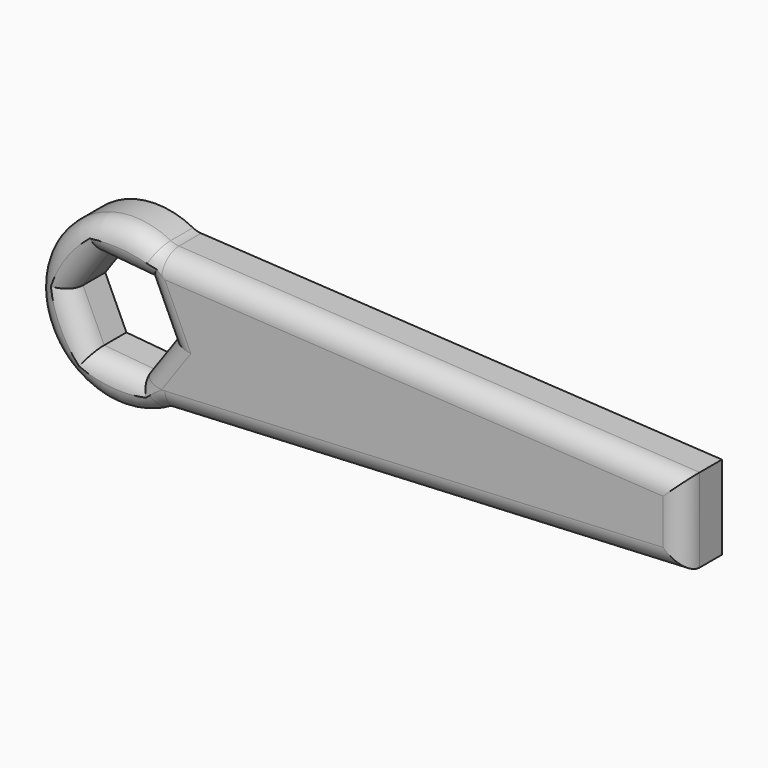
from build123d import *

# Parameters (mm, degrees)
F1_DEPTH      = 11.8
F2_T3_ANGLE   = 23.9952218253
F2_T6_ANGLE   = 236.5757489995
F2_T9_ANGLE   = 26.5092715393
F2_T12_DEPTH  = 139.4367119933
F2_T15_DEPTH  = 45.5289069563
F2_T18_DEPTH  = 140.3160479541
F2_T21_DEPTH  = 37.3901770892
F2_T26_DEPTH  = 37.3901770892
F2_T31_DEPTH  = 37.3901770892
F2_T36_DEPTH  = 37.3901770892
F2_T41_DEPTH  = 37.3901770892
F2_T46_DEPTH  = 37.3901770892
F2_T52_DEPTH  = 37.3901770892
F2_T56_DEPTH  = 37.3901770892
F2_T62_DEPTH  = 37.3901770892
F2_T66_DEPTH  = 37.3901770892
F2_T72_DEPTH  = 37.3901770892
F2_T76_DEPTH  = 37.3901770892
F2_T82_DEPTH  = 37.3901770892
F2_T86_DEPTH  = 37.3901770892
F2_T92_DEPTH  = 37.3901770892
F2_T96_DEPTH  = 37.3901770892
F2_T102_DEPTH = 37.3901770892
F2_T106_DEPTH = 37.3901770892


# Not quite as in the source:
# - a fillet or chamfer that OpenCascade refuses, or shapes differently, is made with other operations: its cross-section is extruded or revolved along the edge and cut away or added


with BuildPart() as f1:
    # F0 (on Front) → F1 (new body)
    with BuildSketch(Plane.XZ):
        with BuildLine():
            ThreePointArc((-45.4681624589, 17.2222085509), (-46.4995658162, 17.3907127083), (-47.4734123647, 17.7699348549))
            ThreePointArc((-47.4734123647, 17.7699348549), (-76.6250444945, -0.3533911925), (-46.8510355825, -17.4349893659))
            ThreePointArc((-46.8510355825, -17.4349893659), (-45.7861203938, -16.9901072457), (-44.6475715962, -16.8012393137))
            Line((-44.6475715962, -16.8012393137), (82.1385234594, -10.6194149703))
            Line((82.1385234594, -10.6194149703), (82.1385234594, 9.909491986))
            Line((82.1385234594, 9.909491986), (-45.4681624589, 17.2222085509))
        make_face()
        Polygon((-49.4849642992, 10.1187057679), (-44.2971102089, -1.1330789012), (-51.4475145251, -11.2517846691), (-63.7857729316, -10.1187057679), (-68.9736270219, 1.1330789012), (-61.8232227057, 11.2517846691), align=None, mode=Mode.SUBTRACT)
    extrude(amount=F1_DEPTH)

    # F2: fillet of radius 5 on 12 edges, made by hand


with BuildPart() as f2_tool1:
    # F2_s2 → F2_t3 (revolve)
    with BuildSketch(Plane(origin=(-46.3030483671, 0, 2.6534743565), x_dir=(0, 1, 0), z_dir=(0.9983620051, 0, -0.0572128202))):
        with BuildLine():
            ThreePointArc((-6.8, 14.5926368593), (-10.3355339059, 13.1281707652), (-11.8, 9.5926368593))
            Line((-11.8, 9.5926368593), (-11.8, 14.5926368593))
            Line((-11.8, 14.5926368593), (-6.8, 14.5926368593))
        make_face()
    revolve(axis=Axis((-45.1820983581, -11.8, 22.2140185763), (0, 1, 0)), revolution_arc=F2_T3_ANGLE)


with BuildPart() as f2_tool4:
    # F2_s5 → F2_t6 (revolve)
    with BuildSketch(Plane(origin=(-44.7416696351, 0, 23.0682455015), x_dir=(0, 1, 0), z_dir=(0.8888167443, 0, -0.4582628013))):
        with BuildLine():
            ThreePointArc((-6.8, -5.9610832949), (-10.3355339059, -7.425549389), (-11.8, -10.9610832949))
            Line((-11.8, -10.9610832949), (-11.8, -5.9610832949))
            Line((-11.8, -5.9610832949), (-6.8, -5.9610832949))
        make_face()
    revolve(axis=Axis((-56.6353686154, -11.8, 0), (0, -1, 0)), revolution_arc=F2_T6_ANGLE)


with BuildPart() as f2_tool7:
    # F2_s8 → F2_t9 (revolve)
    with BuildSketch(Plane(origin=(-43.0708942729, 0, -24.1709337899), x_dir=(0, 1, 0), z_dir=(-0.8720634381, 0, -0.4893928482))):
        with BuildLine():
            ThreePointArc((-6.8, -7.7241449756), (-10.3355339059, -9.1886110696), (-11.8, -12.7241449756))
            Line((-11.8, -12.7241449756), (-11.8, -7.7241449756))
            Line((-11.8, -7.7241449756), (-6.8, -7.7241449756))
        make_face()
    revolve(axis=Axis((-44.4040713414, -11.8, -21.7953065565), (0, 1, 0)), revolution_arc=F2_T9_ANGLE)


with BuildPart() as f2_tool10:
    # F2_s11 → F2_t12 (new body)
    with BuildSketch(Plane(origin=(-45.3589315248, 0, -2.2116064618), x_dir=(0, 1, 0), z_dir=(0.9988134486, 0, 0.048700051))):
        with BuildLine():
            ThreePointArc((-6.8, -14.6069647669), (-10.3355339059, -13.1424986728), (-11.8, -9.6069647669))
            Line((-11.8, -9.6069647669), (-11.8, -14.6069647669))
            Line((-11.8, -14.6069647669), (-6.8, -14.6069647669))
        make_face()
    extrude(amount=F2_T12_DEPTH)


with BuildPart() as f2_tool13:
    # F2_s14 → F2_t15 (new body)
    with BuildSketch(Plane.XY.offset(-23.1194149703)):
        with BuildLine():
            ThreePointArc((82.1385234594, -6.8), (80.6740573654, -10.3355339059), (77.1385234594, -11.8))
            Line((77.1385234594, -11.8), (82.1385234594, -11.8))
            Line((82.1385234594, -11.8), (82.1385234594, -6.8))
        make_face()
    extrude(amount=F2_T15_DEPTH)


with BuildPart() as f2_tool16:
    # F2_s17 → F2_t18 (new body)
    with BuildSketch(Plane(origin=(93.7831626148, 0, -5.3744024604), x_dir=(0, 1, 0), z_dir=(-0.9983620051, 0, 0.0572128202))):
        with BuildLine():
            ThreePointArc((-6.8, -14.5926368593), (-10.3355339059, -13.1281707652), (-11.8, -9.5926368593))
            Line((-11.8, -9.5926368593), (-11.8, -14.5926368593))
            Line((-11.8, -14.5926368593), (-6.8, -14.5926368593))
        make_face()
    extrude(amount=F2_T18_DEPTH)


with BuildPart() as f2_tool19:
    # F2_s20 → F2_t21 (new body)
    with BuildSketch(Plane(origin=(-29.6512532209, 0, -41.9601876654), x_dir=(0, 1, 0), z_dir=(0.5771026729, 0, 0.8166716016))):
        with BuildLine():
            ThreePointArc((-6.8, 56.9827053125), (-10.3355339059, 58.4471714066), (-11.8, 61.9827053125))
            Line((-11.8, 61.9827053125), (-11.8, 56.9827053125))
            Line((-11.8, 56.9827053125), (-6.8, 56.9827053125))
        make_face()
    extrude(amount=F2_T21_DEPTH)

    split(bisect_by=Plane(origin=(-56.450638263, 0, -26.0276643418), x_dir=(0, 1, 0), z_dir=(0.9081213762, 0, 0.4187070171)), keep=Keep.TOP)

    split(bisect_by=Plane(origin=(0.5076300556, 0, 5.5276563658), x_dir=(0, 1, 0), z_dir=(-0.0914497745, 0, -0.99580969)), keep=Keep.TOP)


with BuildPart() as f2_tool24:
    # F2_s25 → F2_t26 (new body)
    with BuildSketch(Plane(origin=(-74.7784738866, 0, 6.867250485), x_dir=(0, 1, 0), z_dir=(0.99580969, 0, -0.0914497745))):
        with BuildLine():
            ThreePointArc((-6.8, 5.5509164263), (-10.3355339059, 7.0153825204), (-11.8, 10.5509164263))
            Line((-11.8, 10.5509164263), (-11.8, 5.5509164263))
            Line((-11.8, 5.5509164263), (-6.8, 5.5509164263))
        make_face()
    extrude(amount=F2_T26_DEPTH)

    split(bisect_by=Plane(origin=(-46.5361572126, 0, 32.8848715463), x_dir=(0, 1, 0), z_dir=(0.8166716016, 0, -0.5771026729)), keep=Keep.TOP)

    split(bisect_by=Plane(origin=(-36.9619755402, 0, -17.0420374751), x_dir=(0, 1, 0), z_dir=(-0.9081213762, 0, -0.4187070171)), keep=Keep.TOP)


with BuildPart() as f2_tool29:
    # F2_s30 → F2_t31 (new body)
    with BuildSketch(Plane(origin=(-17.7568264726, 0, 38.512260445), x_dir=(0, 1, 0), z_dir=(0.4187070171, 0, -0.9081213762))):
        with BuildLine():
            ThreePointArc((-6.8, -40.7015807695), (-10.3355339059, -39.2371146755), (-11.8, -35.7015807695))
            Line((-11.8, -35.7015807695), (-11.8, -40.7015807695))
            Line((-11.8, -40.7015807695), (-6.8, -40.7015807695))
        make_face()
    extrude(amount=F2_T31_DEPTH)

    split(bisect_by=Plane(origin=(0.5076300556, 0, 5.5276563658), x_dir=(0, 1, 0), z_dir=(-0.0914497745, 0, -0.99580969)), keep=Keep.TOP)

    split(bisect_by=Plane(origin=(-29.0100447157, 0, 20.500007976), x_dir=(0, 1, 0), z_dir=(-0.8166716016, 0, 0.5771026729)), keep=Keep.TOP)


with BuildPart() as f2_tool34:
    # F2_s35 → F2_t36 (new body)
    with BuildSketch(Plane(origin=(-8.0732820816, 0, -11.4246918569), x_dir=(0, 1, 0), z_dir=(-0.5771026729, 0, -0.8166716016))):
        with BuildLine():
            ThreePointArc((-6.8, -35.5222890792), (-10.3355339059, -34.0578229851), (-11.8, -30.5222890792))
            Line((-11.8, -30.5222890792), (-11.8, -35.5222890792))
            Line((-11.8, -35.5222890792), (-6.8, -35.5222890792))
        make_face()
    extrude(amount=F2_T36_DEPTH)

    split(bisect_by=Plane(origin=(-36.9619755402, 0, -17.0420374751), x_dir=(0, 1, 0), z_dir=(-0.9081213762, 0, -0.4187070171)), keep=Keep.TOP)

    split(bisect_by=Plane(origin=(-1.4549201703, 0, -15.8428340712), x_dir=(0, 1, 0), z_dir=(0.0914497745, 0, 0.99580969)), keep=Keep.TOP)


with BuildPart() as f2_tool39:
    # F2_s40 → F2_t41 (new body)
    with BuildSketch(Plane(origin=(-37.5449732296, 0, 3.4479272205), x_dir=(0, 1, 0), z_dir=(-0.99580969, 0, 0.0914497745))):
        with BuildLine():
            ThreePointArc((-6.8, 15.909499807), (-10.3355339059, 17.3739659011), (-11.8, 20.909499807))
            Line((-11.8, 20.909499807), (-11.8, 15.909499807))
            Line((-11.8, 15.909499807), (-6.8, 15.909499807))
        make_face()
    extrude(amount=F2_T41_DEPTH)

    split(bisect_by=Plane(origin=(-29.0100447157, 0, 20.500007976), x_dir=(0, 1, 0), z_dir=(-0.8166716016, 0, 0.5771026729)), keep=Keep.TOP)

    split(bisect_by=Plane(origin=(-56.450638263, 0, -26.0276643418), x_dir=(0, 1, 0), z_dir=(0.9081213762, 0, 0.4187070171)), keep=Keep.TOP)


with BuildPart() as f2_tool44:
    # F2_s45 → F2_t46 (new body)
    with BuildSketch(Plane(origin=(-2.1012969549, 0, 4.5574413719), x_dir=(0, 1, 0), z_dir=(-0.4187070171, 0, 0.9081213762))):
        with BuildLine():
            ThreePointArc((-6.8, 62.1619970029), (-10.3355339059, 63.626463097), (-11.8, 67.1619970029))
            Line((-11.8, 67.1619970029), (-11.8, 62.1619970029))
            Line((-11.8, 62.1619970029), (-6.8, 62.1619970029))
        make_face()
    extrude(amount=F2_T46_DEPTH)

    split(bisect_by=Plane(origin=(-46.5361572126, 0, 32.8848715463), x_dir=(0, 1, 0), z_dir=(0.8166716016, 0, -0.5771026729)), keep=Keep.TOP)

    split(bisect_by=Plane(origin=(-1.4549201703, 0, -15.8428340712), x_dir=(0, 1, 0), z_dir=(0.0914497745, 0, 0.99580969)), keep=Keep.TOP)


with BuildPart() as f2_tool50:
    # F2_s51 → F2_t52 (new body)
    with BuildSketch(Plane(origin=(-29.6512532209, 0, -41.9601876654), x_dir=(0, 1, 0), z_dir=(0.5771026729, 0, 0.8166716016))):
        with BuildLine():
            ThreePointArc((-6.8, 56.9827053125), (-10.3355339059, 58.4471714066), (-11.8, 61.9827053125))
            Line((-11.8, 61.9827053125), (-11.8, 56.9827053125))
            Line((-11.8, 56.9827053125), (-6.8, 56.9827053125))
        make_face()
    extrude(amount=F2_T52_DEPTH)

    split(bisect_by=Plane(origin=(-56.450638263, 0, -26.0276643418), x_dir=(0, 1, 0), z_dir=(-0.9081213762, 0, -0.4187070171)), keep=Keep.TOP)


with BuildPart() as f2_tool54:
    # F2_s55 → F2_t56 (new body)
    with BuildSketch(Plane(origin=(-2.1012969549, 0, 4.5574413719), x_dir=(0, 1, 0), z_dir=(-0.4187070171, 0, 0.9081213762))):
        with BuildLine():
            ThreePointArc((-6.8, 62.1619970029), (-10.3355339059, 63.626463097), (-11.8, 67.1619970029))
            Line((-11.8, 67.1619970029), (-11.8, 62.1619970029))
            Line((-11.8, 62.1619970029), (-6.8, 62.1619970029))
        make_face()
    extrude(amount=F2_T56_DEPTH)

    split(bisect_by=Plane(origin=(-46.5361572126, 0, 32.8848715463), x_dir=(0, 1, 0), z_dir=(-0.8166716016, 0, 0.5771026729)), keep=Keep.TOP)


with BuildPart() as f2_tool50_1:
    add(f2_tool50.part)

    # F2_t58: intersect F2_tool54
    add(f2_tool54.part, mode=Mode.INTERSECT)


with BuildPart() as f2_tool60:
    # F2_s61 → F2_t62 (new body)
    with BuildSketch(Plane(origin=(-29.6512532209, 0, -41.9601876654), x_dir=(0, 1, 0), z_dir=(0.5771026729, 0, 0.8166716016))):
        with BuildLine():
            ThreePointArc((-6.8, 56.9827053125), (-10.3355339059, 58.4471714066), (-11.8, 61.9827053125))
            Line((-11.8, 61.9827053125), (-11.8, 56.9827053125))
            Line((-11.8, 56.9827053125), (-6.8, 56.9827053125))
        make_face()
    extrude(amount=F2_T62_DEPTH)

    split(bisect_by=Plane(origin=(0.5076300556, 0, 5.5276563658), x_dir=(0, 1, 0), z_dir=(0.0914497745, 0, 0.99580969)), keep=Keep.TOP)


with BuildPart() as f2_tool64:
    # F2_s65 → F2_t66 (new body)
    with BuildSketch(Plane(origin=(-74.7784738866, 0, 6.867250485), x_dir=(0, 1, 0), z_dir=(0.99580969, 0, -0.0914497745))):
        with BuildLine():
            ThreePointArc((-6.8, 5.5509164263), (-10.3355339059, 7.0153825204), (-11.8, 10.5509164263))
            Line((-11.8, 10.5509164263), (-11.8, 5.5509164263))
            Line((-11.8, 5.5509164263), (-6.8, 5.5509164263))
        make_face()
    extrude(amount=F2_T66_DEPTH)

    split(bisect_by=Plane(origin=(-46.5361572126, 0, 32.8848715463), x_dir=(0, 1, 0), z_dir=(-0.8166716016, 0, 0.5771026729)), keep=Keep.TOP)


with BuildPart() as f2_tool60_1:
    add(f2_tool60.part)

    # F2_t68: intersect F2_tool64
    add(f2_tool64.part, mode=Mode.INTERSECT)


with BuildPart() as f2_tool70:
    # F2_s71 → F2_t72 (new body)
    with BuildSketch(Plane(origin=(-74.7784738866, 0, 6.867250485), x_dir=(0, 1, 0), z_dir=(0.99580969, 0, -0.0914497745))):
        with BuildLine():
            ThreePointArc((-6.8, 5.5509164263), (-10.3355339059, 7.0153825204), (-11.8, 10.5509164263))
            Line((-11.8, 10.5509164263), (-11.8, 5.5509164263))
            Line((-11.8, 5.5509164263), (-6.8, 5.5509164263))
        make_face()
    extrude(amount=F2_T72_DEPTH)

    split(bisect_by=Plane(origin=(-36.9619755402, 0, -17.0420374751), x_dir=(0, 1, 0), z_dir=(0.9081213762, 0, 0.4187070171)), keep=Keep.TOP)


with BuildPart() as f2_tool74:
    # F2_s75 → F2_t76 (new body)
    with BuildSketch(Plane(origin=(-17.7568264726, 0, 38.512260445), x_dir=(0, 1, 0), z_dir=(0.4187070171, 0, -0.9081213762))):
        with BuildLine():
            ThreePointArc((-6.8, -40.7015807695), (-10.3355339059, -39.2371146755), (-11.8, -35.7015807695))
            Line((-11.8, -35.7015807695), (-11.8, -40.7015807695))
            Line((-11.8, -40.7015807695), (-6.8, -40.7015807695))
        make_face()
    extrude(amount=F2_T76_DEPTH)

    split(bisect_by=Plane(origin=(0.5076300556, 0, 5.5276563658), x_dir=(0, 1, 0), z_dir=(0.0914497745, 0, 0.99580969)), keep=Keep.TOP)


with BuildPart() as f2_tool70_1:
    add(f2_tool70.part)

    # F2_t78: intersect F2_tool74
    add(f2_tool74.part, mode=Mode.INTERSECT)


with BuildPart() as f2_tool80:
    # F2_s81 → F2_t82 (new body)
    with BuildSketch(Plane(origin=(-17.7568264726, 0, 38.512260445), x_dir=(0, 1, 0), z_dir=(0.4187070171, 0, -0.9081213762))):
        with BuildLine():
            ThreePointArc((-6.8, -40.7015807695), (-10.3355339059, -39.2371146755), (-11.8, -35.7015807695))
            Line((-11.8, -35.7015807695), (-11.8, -40.7015807695))
            Line((-11.8, -40.7015807695), (-6.8, -40.7015807695))
        make_face()
    extrude(amount=F2_T82_DEPTH)

    split(bisect_by=Plane(origin=(-29.0100447157, 0, 20.500007976), x_dir=(0, 1, 0), z_dir=(0.8166716016, 0, -0.5771026729)), keep=Keep.TOP)


with BuildPart() as f2_tool84:
    # F2_s85 → F2_t86 (new body)
    with BuildSketch(Plane(origin=(-8.0732820816, 0, -11.4246918569), x_dir=(0, 1, 0), z_dir=(-0.5771026729, 0, -0.8166716016))):
        with BuildLine():
            ThreePointArc((-6.8, -35.5222890792), (-10.3355339059, -34.0578229851), (-11.8, -30.5222890792))
            Line((-11.8, -30.5222890792), (-11.8, -35.5222890792))
            Line((-11.8, -35.5222890792), (-6.8, -35.5222890792))
        make_face()
    extrude(amount=F2_T86_DEPTH)

    split(bisect_by=Plane(origin=(-36.9619755402, 0, -17.0420374751), x_dir=(0, 1, 0), z_dir=(0.9081213762, 0, 0.4187070171)), keep=Keep.TOP)


with BuildPart() as f2_tool80_1:
    add(f2_tool80.part)

    # F2_t88: intersect F2_tool84
    add(f2_tool84.part, mode=Mode.INTERSECT)


with BuildPart() as f2_tool90:
    # F2_s91 → F2_t92 (new body)
    with BuildSketch(Plane(origin=(-8.0732820816, 0, -11.4246918569), x_dir=(0, 1, 0), z_dir=(-0.5771026729, 0, -0.8166716016))):
        with BuildLine():
            ThreePointArc((-6.8, -35.5222890792), (-10.3355339059, -34.0578229851), (-11.8, -30.5222890792))
            Line((-11.8, -30.5222890792), (-11.8, -35.5222890792))
            Line((-11.8, -35.5222890792), (-6.8, -35.5222890792))
        make_face()
    extrude(amount=F2_T92_DEPTH)

    split(bisect_by=Plane(origin=(-1.4549201703, 0, -15.8428340712), x_dir=(0, 1, 0), z_dir=(-0.0914497745, 0, -0.99580969)), keep=Keep.TOP)


with BuildPart() as f2_tool94:
    # F2_s95 → F2_t96 (new body)
    with BuildSketch(Plane(origin=(-37.5449732296, 0, 3.4479272205), x_dir=(0, 1, 0), z_dir=(-0.99580969, 0, 0.0914497745))):
        with BuildLine():
            ThreePointArc((-6.8, 15.909499807), (-10.3355339059, 17.3739659011), (-11.8, 20.909499807))
            Line((-11.8, 20.909499807), (-11.8, 15.909499807))
            Line((-11.8, 15.909499807), (-6.8, 15.909499807))
        make_face()
    extrude(amount=F2_T96_DEPTH)

    split(bisect_by=Plane(origin=(-29.0100447157, 0, 20.500007976), x_dir=(0, 1, 0), z_dir=(0.8166716016, 0, -0.5771026729)), keep=Keep.TOP)


with BuildPart() as f2_tool90_1:
    add(f2_tool90.part)

    # F2_t98: intersect F2_tool94
    add(f2_tool94.part, mode=Mode.INTERSECT)


with BuildPart() as f2_tool100:
    # F2_s101 → F2_t102 (new body)
    with BuildSketch(Plane(origin=(-37.5449732296, 0, 3.4479272205), x_dir=(0, 1, 0), z_dir=(-0.99580969, 0, 0.0914497745))):
        with BuildLine():
            ThreePointArc((-6.8, 15.909499807), (-10.3355339059, 17.3739659011), (-11.8, 20.909499807))
            Line((-11.8, 20.909499807), (-11.8, 15.909499807))
            Line((-11.8, 15.909499807), (-6.8, 15.909499807))
        make_face()
    extrude(amount=F2_T102_DEPTH)

    split(bisect_by=Plane(origin=(-56.450638263, 0, -26.0276643418), x_dir=(0, 1, 0), z_dir=(-0.9081213762, 0, -0.4187070171)), keep=Keep.TOP)


with BuildPart() as f2_tool104:
    # F2_s105 → F2_t106 (new body)
    with BuildSketch(Plane(origin=(-2.1012969549, 0, 4.5574413719), x_dir=(0, 1, 0), z_dir=(-0.4187070171, 0, 0.9081213762))):
        with BuildLine():
            ThreePointArc((-6.8, 62.1619970029), (-10.3355339059, 63.626463097), (-11.8, 67.1619970029))
            Line((-11.8, 67.1619970029), (-11.8, 62.1619970029))
            Line((-11.8, 62.1619970029), (-6.8, 62.1619970029))
        make_face()
    extrude(amount=F2_T106_DEPTH)

    split(bisect_by=Plane(origin=(-1.4549201703, 0, -15.8428340712), x_dir=(0, 1, 0), z_dir=(-0.0914497745, 0, -0.99580969)), keep=Keep.TOP)


with BuildPart() as f2_tool100_1:
    add(f2_tool100.part)

    # F2_t108: intersect F2_tool104
    add(f2_tool104.part, mode=Mode.INTERSECT)


with BuildPart() as f1_1:
    add(f1.part)

    # F2_t109: cut F2_tool1, F2_tool4, F2_tool7, F2_tool10, F2_tool13, F2_tool16, F2_tool19, F2_tool24, F2_tool29, F2_tool34, F2_tool39, F2_tool44, F2_tool50, F2_tool60, F2_tool70, F2_tool80, F2_tool90, F2_tool100
    add([f2_tool1.part, f2_tool4.part, f2_tool7.part, f2_tool10.part, f2_tool13.part, f2_tool16.part, f2_tool19.part, f2_tool24.part, f2_tool29.part, f2_tool34.part, f2_tool39.part, f2_tool44.part, f2_tool50_1.part, f2_tool60_1.part, f2_tool70_1.part, f2_tool80_1.part, f2_tool90_1.part, f2_tool100_1.part], mode=Mode.SUBTRACT)


solid = f1_1.part
